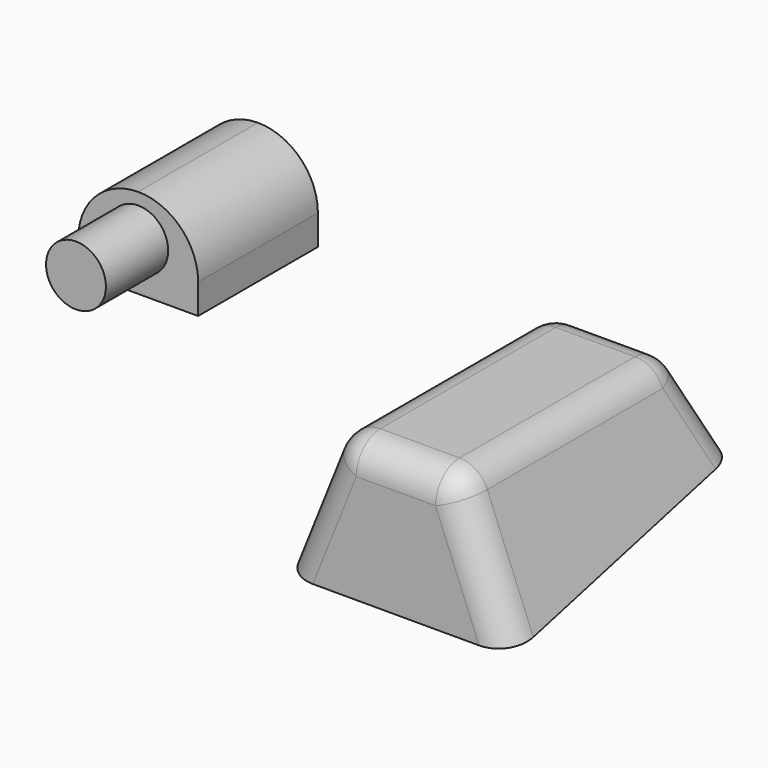
from build123d import *

# Parameters (mm, degrees)
F0_W        = 40
F0_H        = 55
F1_DEPTH    = 25
F2_T1_DEPTH = 383.0272640249
F3_T1_DEPTH = 184.6556819565
F3_T3_DEPTH = 169.6556819565
F4_R        = 5
F5_T        = -2
F0_W_2      = 20
F0_H_2      = 25
F6_DEPTH    = 15
F7_R        = 9.99999
F8_R        = 5
F9_DEPTH    = 13


# Not quite as in the source:
# - a fillet or chamfer that OpenCascade refuses, or shapes differently, is made with other operations: its cross-section is extruded or revolved along the edge and cut away or added
# - a fillet or chamfer is up to 0.001 mm smaller than in the source, because OpenCascade refuses the exact size


with BuildPart() as f1:
    # F0 (on Top) → F1 (new body)
    with BuildSketch(Plane.XY):
        Rectangle(F0_W, F0_H)
    extrude(amount=-F1_DEPTH)

    # F2: chamfer of 11 x 66 on 1 edges, made by hand

    # F2_s2 → F2_t1 (cut)
    with BuildSketch(Plane.YZ.offset(-191.5136320125)):
        Polygon((27.5, -14), (-38.5, -25), (27.5, -25), align=None)
    extrude(amount=F2_T1_DEPTH, mode=Mode.SUBTRACT)

    # F3: chamfer of 10 x 25 on 3 edges, made by hand

    # F3_s2 → F3_t1 (cut)
    with BuildSketch(Plane.XZ.offset(-92.3278409783)):
        Polygon((10, 0), (20, -25), (20, 0), align=None)
        Polygon((-20, -25), (-10, 0), (-20, 0), align=None)
    extrude(amount=F3_T1_DEPTH, mode=Mode.SUBTRACT)

    # F3_s4 → F3_t3 (cut)
    with BuildSketch(Plane.YZ.offset(-84.8278409783)):
        Polygon((17.5, 0), (27.5, -25), (27.5, 0), align=None)
    extrude(amount=F3_T3_DEPTH, mode=Mode.SUBTRACT)

    # F4
    f4_edges = [f1.edges().sort_by_distance(p)[0] for p in [
        (10, -5, 0),
        (0, -27.5, 0),
        (-10, -5, 0),
        (0, 17.5, 0),
        (-12.9375, 20.4375, -7.34375),
        (12.9375, 20.4375, -7.34375),
        (-14.633333, -27.5, -11.583333),
        (14.633333, -27.5, -11.583333),
    ]]
    fillet(f4_edges, radius=F4_R)

    # F5
    f5_openings = [f1.faces().sort_by_distance(p)[0] for p in [
        (0, -2.846063, -19.057677),
    ]]
    offset(amount=F5_T, openings=f5_openings)


with BuildPart() as f6:
    # F0 (on Top) → F6 (new body)
    with BuildSketch(Plane.XY):
        with Locations((-55.0338290632, 0)):
            Rectangle(F0_W_2, F0_H_2)
    extrude(amount=F6_DEPTH)

    # F7 (radius 10 in the source; OpenCascade refuses exactly that, so slightly less here)
    f7_edges = [f6.edges().sort_by_distance(p)[0] for p in [
        (-45.033829, 0, 15),
        (-65.033829, 0, 15),
    ]]
    fillet(f7_edges, radius=F7_R)

    # F8 (on face) → F9 (join)
    with BuildSketch(Plane.XZ.offset(12.5)):
        with Locations((-55.0338290632, 8)):
            Circle(F8_R)
    extrude(amount=F9_DEPTH)


solid = Compound([f1.part, f6.part])
